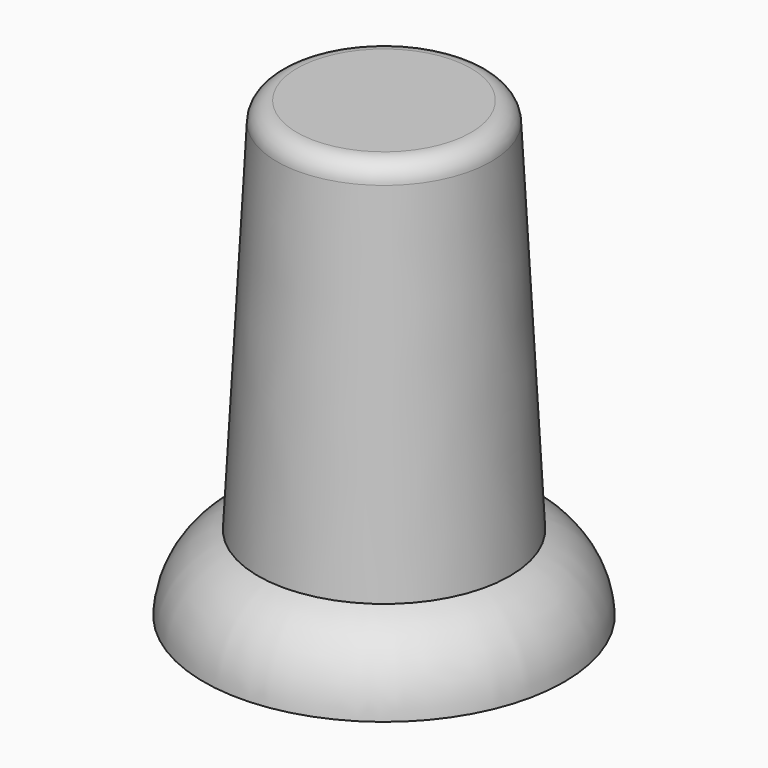
from build123d import *

# Parameters (mm, degrees)
F0_R     = 5
F1_DEPTH = 15
F1_TAPER = 3
F0_R_2   = 7
F2_DEPTH = 4
F2_TAPER = 3
F3_R     = 0.8
F5_DEPTH = 3
F5_TAPER = -3


# Not quite as in the source:
# - a fillet or chamfer that OpenCascade refuses, or shapes differently, is made with other operations: its cross-section is extruded or revolved along the edge and cut away or added


with BuildPart() as f1:
    # F0 (on Top) → F1 (new body)
    with BuildSketch(Plane.XY):
        with Locations((-26.8780887127, 32.4224531651)):
            Circle(F0_R)
    extrude(amount=F1_DEPTH, taper=F1_TAPER)

    # F3
    f3_edges = [f1.edges().sort_by_distance(p)[0] for p in [
        (-31.091972, 32.422453, 15),
    ]]
    fillet(f3_edges, radius=F3_R)


with BuildPart() as f2:
    # F0 (on Top) → F2 (new body)
    with BuildSketch(Plane.XY):
        with Locations((-26.8780887127, 32.4224531651)):
            Circle(F0_R_2)
        with Locations((-26.8780887127, 32.4224531651)):
            Circle(F0_R, mode=Mode.SUBTRACT)
    extrude(amount=F2_DEPTH, taper=F2_TAPER)


with BuildPart() as f5:
    # F0 (on Top) → F5 (new body)
    with BuildSketch(Plane.XY):
        with Locations((-26.8780887127, 32.4224531651)):
            Circle(F0_R_2)
        with Locations((-26.8780887127, 32.4224531651)):
            Circle(F0_R, mode=Mode.SUBTRACT)
    extrude(amount=-F5_DEPTH, taper=F5_TAPER)

    # F6: fillet of radius 3.4 on 1 edges, made by hand

    # F6_s1 → F6_t2 (revolve, cut)
    with BuildSketch(Plane.XZ.offset(-32.4224531651)):
        with BuildLine():
            ThreePointArc((-19.7214746815, -2.9883737372), (-20.3597807896, -1.1766522446), (-21.8780887127, 0))
            Line((-21.8780887127, 0), (-21.853314185, 0.0633263198))
            ThreePointArc((-21.853314185, 0.0633263198), (-20.8780887127, 0.068), (-19.8780887127, 0.068))
            Line((-19.8780887127, 0.068), (-19.8101819043, 0.003558845))
            Line((-19.8101819043, 0.003558845), (-19.6535678731, -2.9848148921))
            Line((-19.6535678731, -2.9848148921), (-19.7214746815, -2.9883737372))
        make_face()
    revolve(axis=Axis((-26.8780887127, 32.4224531651, 0), (0, 0, -1)), mode=Mode.SUBTRACT)


solid = Compound([f1.part, f5.part])
